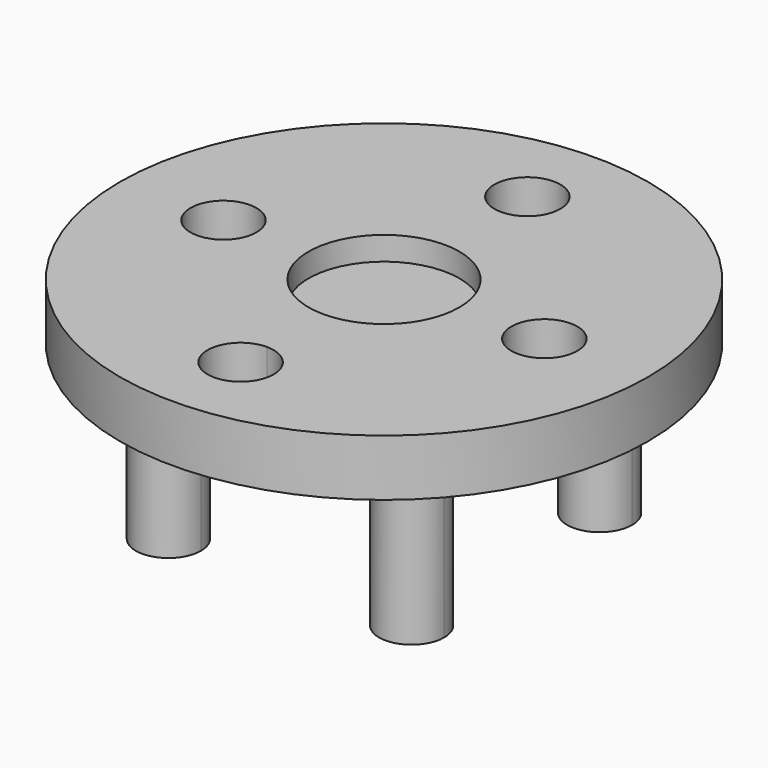
from build123d import *

# Parameters (mm, degrees)
F0_R     = 14
F1_DEPTH = 3
F2_R     = 4
F3_DEPTH = 1.25
F5_DEPTH = 11.5
F6_DEPTH = 25.4
F4_R     = 1.75
F7_DEPTH = 25.4


# Not quite as in the source:
# - a feature names something its author has since deleted; it is built from what else it names


with BuildPart() as f1:
    # F0 (on Top) → F1 (new body)
    with BuildSketch(Plane.XY):
        with Locations((-41.5364727378, -7.5015998445)):
            Circle(F0_R)
    extrude(amount=F1_DEPTH)

    # F2 (on face) → F3 (cut)
    with BuildSketch(Plane.XY.offset(3)):
        with Locations((-41.5364727378, -7.5015998445)):
            Circle(F2_R)
    extrude(amount=-F3_DEPTH, mode=Mode.SUBTRACT)

    # F4 (on face) → F5 (join)
    with BuildSketch(Plane.XY.offset(3)):
        with BuildLine():
            ThreePointArc((-46.2922708097, -1.256661386), (-49.6170112359, -0.6113276981), (-46.7751178459, -2.4536079239))
            ThreePointArc((-46.7751178459, -2.4536079239), (-46.4175303835, -1.9019950739), (-46.2922708097, -1.256661386))
        make_face()
        with BuildLine():
            ThreePointArc((-33.3423393435, -13.758620951), (-34.4205133346, -12.1594833352), (-36.3072565774, -12.5593585722))
            ThreePointArc((-36.3072565774, -12.5593585722), (-35.7141653523, -15.3577585668), (-33.3423393435, -13.758620951))
        make_face()
        with BuildLine():
            ThreePointArc((-46.0564111963, -13.9823979165), (-46.193904066, -13.3075304398), (-46.5844646585, -12.7402449527))
            ThreePointArc((-46.5844646585, -12.7402449527), (-49.3689183267, -14.6572653931), (-46.0564111963, -13.9823979165))
        make_face()
        with BuildLine():
            ThreePointArc((-33.5665342792, -1.0208017726), (-35.9664017559, 0.5667053577), (-36.4884808171, -2.2629547364))
            ThreePointArc((-36.4884808171, -2.2629547364), (-34.6166668026, -2.608308903), (-33.5665342792, -1.0208017726))
        make_face()
    extrude(amount=-F5_DEPTH)

    # F4 (on face) → F6 (cut)
    with BuildSketch(Plane.XY.offset(3)):
        with BuildLine():
            ThreePointArc((-39.7864727378, 1.9984001555), (-42.7739096049, 3.2358370225), (-41.5364727378, 0.2484001555))
            ThreePointArc((-41.5364727378, 0.2484001555), (-40.2990358707, 0.7609632884), (-39.7864727378, 1.9984001555))
        make_face()
        with BuildLine():
            ThreePointArc((-31.2864727378, -7.5015998445), (-33.0364727378, -5.7515998445), (-34.7864727378, -7.5015998445))
            ThreePointArc((-34.7864727378, -7.5015998445), (-33.0364727378, -9.2515998445), (-31.2864727378, -7.5015998445))
        make_face()
        with BuildLine():
            ThreePointArc((-39.7864727378, -17.0011998445), (-40.2990358707, -15.7637629775), (-41.5364727378, -15.2511998445))
            ThreePointArc((-41.5364727378, -15.2511998445), (-42.7739096049, -18.2386367116), (-39.7864727378, -17.0011998445))
        make_face()
    extrude(amount=-F6_DEPTH, mode=Mode.SUBTRACT)

    # F4 (on face) → F7 (cut)
    with BuildSketch(Plane.XY.offset(3)):
        with Locations((-50.0454727378, -7.5015998445)):
            Circle(F4_R)
    extrude(amount=-F7_DEPTH, mode=Mode.SUBTRACT)


solid = f1.part
